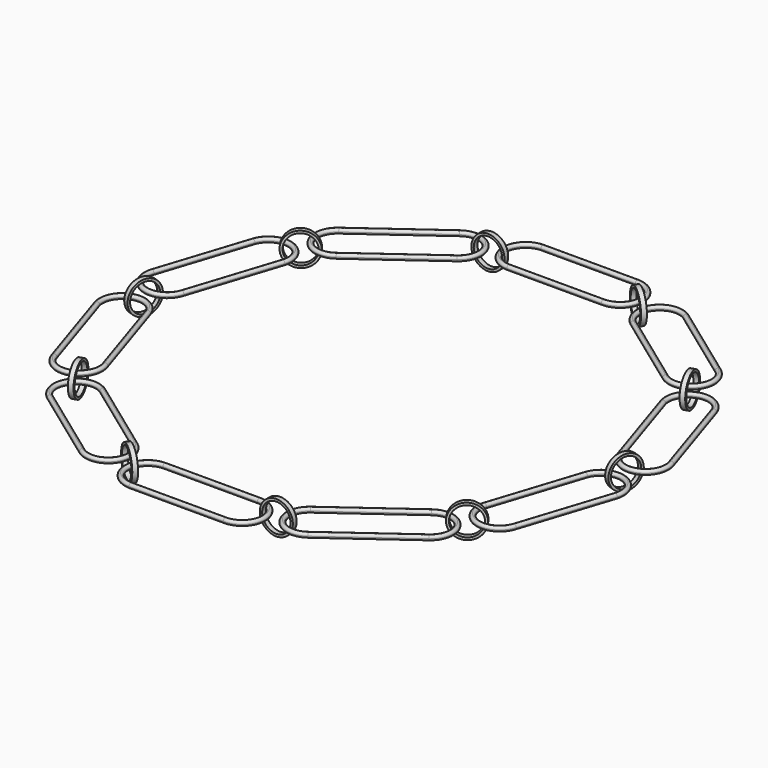
from build123d import *

# Parameters (mm, degrees)
F1_DEPTH = 1
F2_R     = 0.49999
F4_R     = 3.5
F4_R_2   = 3
F5_DEPTH = 0.5
F7_COUNT = 10


# Not quite as in the source:
# - a fillet or chamfer is up to 0.001 mm smaller than in the source, because OpenCascade refuses the exact size


with BuildPart() as f1:
    # F0 (on Top) → F1 (new body)
    with BuildSketch(Plane.XY):
        with BuildLine():
            Line((10, -45), (-10, -45))
            ThreePointArc((-10, -45), (-15, -50), (-10, -55))
            Line((-10, -55), (10, -55))
            ThreePointArc((10, -55), (15, -50), (10, -45))
        make_face()
        with BuildLine():
            ThreePointArc((-10, -53.9999999106), (-13.9999999106, -50), (-10, -46.0000000894))
            Line((-10, -46.0000000894), (10, -46.0000000894))
            ThreePointArc((10, -46.0000000894), (13.9999999106, -50), (10, -53.9999999106))
            Line((10, -53.9999999106), (-10, -53.9999999106))
        make_face(mode=Mode.SUBTRACT)
    extrude(amount=F1_DEPTH)

    # F2 (radius 0.5 in the source; OpenCascade refuses exactly that, so slightly less here)
    f2_edges = [f1.edges().sort_by_distance(p)[0] for p in [
        (0, -45, 0),
        (-15, -50, 0),
        (0, -55, 0),
        (15, -50, 0),
        (-14, -50, 0),
        (0, -46, 0),
        (14, -50, 0),
        (0, -54, 0),
        (0, -45, 1),
        (-15, -50, 1),
        (0, -55, 1),
        (15, -50, 1),
        (-14, -50, 1),
        (0, -46, 1),
        (14, -50, 1),
        (0, -54, 1),
    ]]
    fillet(f2_edges, radius=F2_R)


with BuildPart() as f5:
    # F4 (on offset) → F5 (new body, symmetric)
    with BuildSketch(Plane.XZ.offset(48)):
        with Locations((16, 0.5)):
            Circle(F4_R)
        with Locations((16, 0.5)):
            Circle(F4_R_2, mode=Mode.SUBTRACT)
    extrude(amount=F5_DEPTH, both=True)


with BuildPart() as f7_1:
    # F7: instance of F1
    add(f1.part.rotate(Axis((0, 0, 0.8402345702), (0, 0, -1)), 1 * 360 / F7_COUNT))


with BuildPart() as f7_2:
    # F7: instance of F1
    add(f1.part.rotate(Axis((0, 0, 0.8402345702), (0, 0, -1)), 2 * 360 / F7_COUNT))


with BuildPart() as f7_3:
    # F7: instance of F1
    add(f1.part.rotate(Axis((0, 0, 0.8402345702), (0, 0, -1)), 3 * 360 / F7_COUNT))


with BuildPart() as f7_4:
    # F7: instance of F1
    add(f1.part.rotate(Axis((0, 0, 0.8402345702), (0, 0, -1)), 4 * 360 / F7_COUNT))


with BuildPart() as f7_5:
    # F7: instance of F1
    add(f1.part.rotate(Axis((0, 0, 0.8402345702), (0, 0, -1)), 5 * 360 / F7_COUNT))


with BuildPart() as f7_6:
    # F7: instance of F1
    add(f1.part.rotate(Axis((0, 0, 0.8402345702), (0, 0, -1)), 6 * 360 / F7_COUNT))


with BuildPart() as f7_7:
    # F7: instance of F1
    add(f1.part.rotate(Axis((0, 0, 0.8402345702), (0, 0, -1)), 7 * 360 / F7_COUNT))


with BuildPart() as f7_8:
    # F7: instance of F1
    add(f1.part.rotate(Axis((0, 0, 0.8402345702), (0, 0, -1)), 8 * 360 / F7_COUNT))


with BuildPart() as f7_9:
    # F7: instance of F1
    add(f1.part.rotate(Axis((0, 0, 0.8402345702), (0, 0, -1)), 9 * 360 / F7_COUNT))


with BuildPart() as f7_10:
    # F7: instance of F5
    add(f5.part.rotate(Axis((0, 0, 0.8402345702), (0, 0, -1)), 1 * 360 / F7_COUNT))


with BuildPart() as f7_11:
    # F7: instance of F5
    add(f5.part.rotate(Axis((0, 0, 0.8402345702), (0, 0, -1)), 2 * 360 / F7_COUNT))


with BuildPart() as f7_12:
    # F7: instance of F5
    add(f5.part.rotate(Axis((0, 0, 0.8402345702), (0, 0, -1)), 3 * 360 / F7_COUNT))


with BuildPart() as f7_13:
    # F7: instance of F5
    add(f5.part.rotate(Axis((0, 0, 0.8402345702), (0, 0, -1)), 4 * 360 / F7_COUNT))


with BuildPart() as f7_14:
    # F7: instance of F5
    add(f5.part.rotate(Axis((0, 0, 0.8402345702), (0, 0, -1)), 5 * 360 / F7_COUNT))


with BuildPart() as f7_15:
    # F7: instance of F5
    add(f5.part.rotate(Axis((0, 0, 0.8402345702), (0, 0, -1)), 6 * 360 / F7_COUNT))


with BuildPart() as f7_16:
    # F7: instance of F5
    add(f5.part.rotate(Axis((0, 0, 0.8402345702), (0, 0, -1)), 7 * 360 / F7_COUNT))


with BuildPart() as f7_17:
    # F7: instance of F5
    add(f5.part.rotate(Axis((0, 0, 0.8402345702), (0, 0, -1)), 8 * 360 / F7_COUNT))


with BuildPart() as f7_18:
    # F7: instance of F5
    add(f5.part.rotate(Axis((0, 0, 0.8402345702), (0, 0, -1)), 9 * 360 / F7_COUNT))


solid = Compound([f1.part, f5.part, f7_1.part, f7_2.part, f7_3.part, f7_4.part, f7_5.part, f7_6.part, f7_7.part, f7_8.part, f7_9.part, f7_10.part, f7_11.part, f7_12.part, f7_13.part, f7_14.part, f7_15.part, f7_16.part, f7_17.part, f7_18.part])
